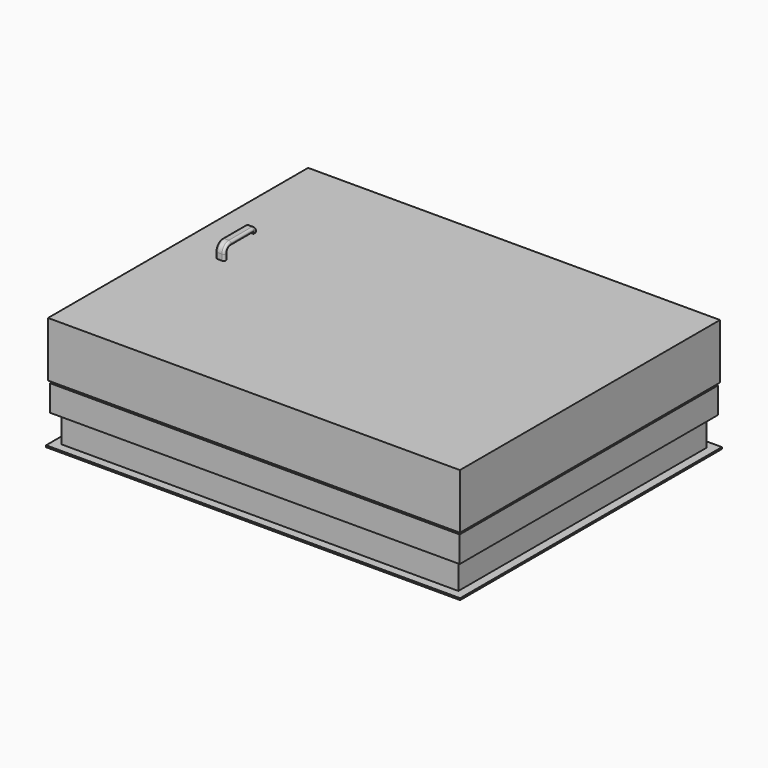
from build123d import *

# Parameters (mm, degrees)
F1_DEPTH = 754
F3_DEPTH = 999
F6_W     = 20
F6_H     = 10
F8_R     = 4.99999
F9_R     = 3


# Not quite as in the source:
# - a fillet or chamfer is up to 0.001 mm smaller than in the source, because OpenCascade refuses the exact size


with BuildPart() as f1:
    # F0 (on Front) → F1 (new body)
    with BuildSketch(Plane.XZ):
        Polygon((-477, -127), (-477, -131), (477, -131), (477, -127), (457, -127), (457, -61.5), (472, -61.5), (472, -1.5), (422, -1.5), (422, 4), (474.5, 4), (474.5, 131), (-474.5, 131), (-474.5, 4), (-422, 4), (-422, -1.5), (-472, -1.5), (-472, -61.5), (-457, -61.5), (-457, -127), align=None)
    extrude(amount=F1_DEPTH)

    # F2 (on face) → F3 (cut)
    with BuildSketch(Plane(origin=(-474.5, 0, 0), x_dir=(0, -1, 0), z_dir=(-1, 0, 0))):
        Polygon((754, -127), (754, -131), (765.5175328255, -131), (774.4438648224, 131), (751.5, 131), (751.5, 4), (699, 4), (699, -1.5), (749, -1.5), (749, -61.5), (734, -61.5), (734, -127), align=None)
        Polygon((55, 4), (2.5, 4), (2.5, 131), (-20.4438648224, 131), (-11.5175328255, -131), (0, -131), (0, -127), (20, -127), (20, -61.5), (5, -61.5), (5, -1.5), (55, -1.5), align=None)
    extrude(amount=-F3_DEPTH, mode=Mode.SUBTRACT)

    # F7: sweep along a path in F5
    with BuildLine(Plane(origin=(-374.5, 0, 0), x_dir=(0, -1, 0), z_dir=(-1, 0, 0))) as f7_path:
        Line((377, 131), (377, 144.4709453487))
        ThreePointArc((377, 144.4709453487), (372.6066017178, 155.0775470665), (362, 159.4709453487))
        Line((362, 159.4709453487), (297, 159.4709453487))
        ThreePointArc((297, 159.4709453487), (293.4644660941, 158.0064792547), (292, 154.4709453487))
        Line((292, 154.4709453487), (292, 150.8713660145))
    # F6 (on face) → F7 (sweep)
    with BuildSketch(Plane.XY.offset(131)):
        with Locations((-374.5, -377)):
            Rectangle(F6_W, F6_H)
    sweep(path=f7_path.line)

    # F8 (radius 5 in the source; OpenCascade refuses exactly that, so slightly less here)
    f8_edges = [f1.edges().sort_by_distance(p)[0] for p in [
        (-384.5, -329.5, 164.470945),
        (-384.5, -329.5, 154.470945),
        (-364.5, -329.5, 164.470945),
        (-364.5, -329.5, 154.470945),
    ]]
    fillet(f8_edges, radius=F8_R)

    # F9
    f9_edges = [f1.edges().sort_by_distance(p)[0] for p in [
        (-374.5, -287, 150.871366),
        (-374.5, -297, 150.871366),
        (-384.5, -294.499995, 150.871366),
    ]]
    fillet(f9_edges, radius=F9_R)


solid = f1.part
